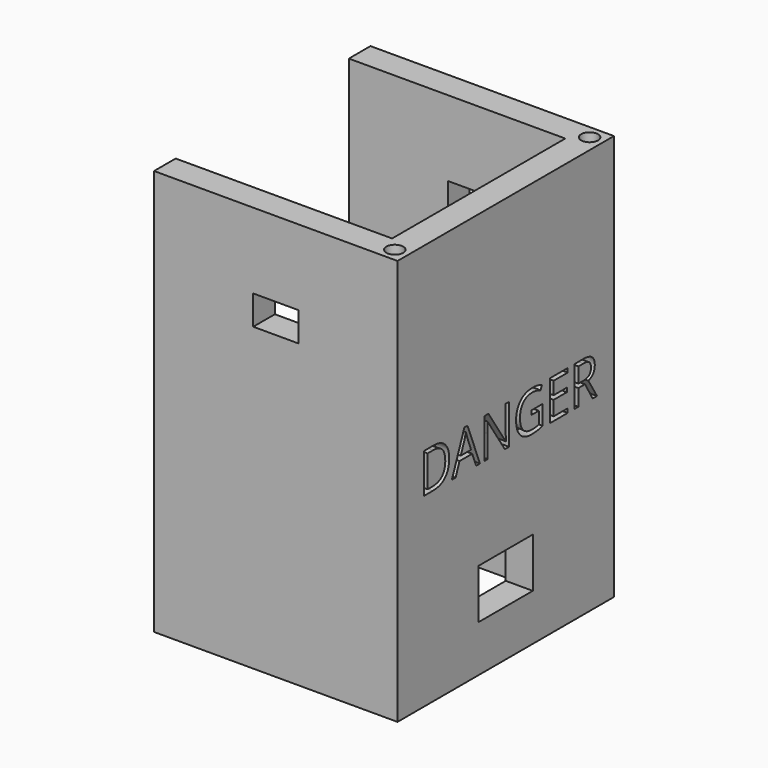
from build123d import *

# Parameters (mm, degrees)
F1_DEPTH      = 90
F2_R          = 1.875
F3_DEPTH      = 9
F4_R          = 1.875
F5_DEPTH      = 9
F6_W          = 10
F6_H          = 6.5
F7_DEPTH      = 6
F8_W          = 10
F8_H          = 6.5
F9_DEPTH      = 6
F10_TEXT_SIZE = 12.2977595019
F11_DEPTH     = 3
F12_W         = 15
F12_H         = 11
F13_DEPTH     = 6


# Not quite as in the source:
# - Text() gives the source's letters only with a copy of the font that has no kerning and outlines rounded to 1/6400 em; it was checked with that copy


with BuildPart() as f1:
    # F0 (on Top) → F1 (new body)
    with BuildSketch(Plane.XY):
        Polygon((27, 30), (-27, 30), (-27, 24), (21, 24), (21, -24), (-27, -24), (-27, -30), (27, -30), (27, 24), align=None)
    extrude(amount=F1_DEPTH)

    # F2 (on face) → F3 (cut)
    with BuildSketch(Plane.XY.offset(90)):
        with Locations((24, 27)):
            Circle(F2_R)
        with Locations((24, -27)):
            Circle(F2_R)
    extrude(amount=-F3_DEPTH, mode=Mode.SUBTRACT)

    # F4 (on face) → F5 (cut)
    with BuildSketch(Plane(origin=(0, 0, 0), x_dir=(1, 0, 0), z_dir=(0, 0, -1))):
        with Locations((24, -27)):
            Circle(F4_R)
        with Locations((24, 27)):
            Circle(F4_R)
    extrude(amount=-F5_DEPTH, mode=Mode.SUBTRACT)

    # F6 (on face) → F7 (cut)
    with BuildSketch(Plane.XZ.offset(30)):
        with Locations((0, 70)):
            Rectangle(F6_W, F6_H)
    extrude(amount=-F7_DEPTH, mode=Mode.SUBTRACT)

    # F8 (on face) → F9 (cut)
    with BuildSketch(Plane(origin=(0, 30, 0), x_dir=(-1, 0, 0), z_dir=(0, 1, 0))):
        with Locations((0, 70)):
            Rectangle(F8_W, F8_H)
    extrude(amount=-F9_DEPTH, mode=Mode.SUBTRACT)

    # F10 (on face) → F11 (cut)
    with BuildSketch(Plane.YZ.offset(27)):
        with Locations((-23.8986311526, 41.1456131586)):
            Text('DANGER', F10_TEXT_SIZE, font='Open Sans', text_align=(TextAlign.LEFT, TextAlign.BOTTOM))
    extrude(amount=-F11_DEPTH, mode=Mode.SUBTRACT)

    # F12 (on face) → F13 (cut)
    with BuildSketch(Plane.YZ.offset(27)):
        with Locations((0, 15.8482156694)):
            Rectangle(F12_W, F12_H)
    extrude(amount=-F13_DEPTH, mode=Mode.SUBTRACT)


solid = f1.part
